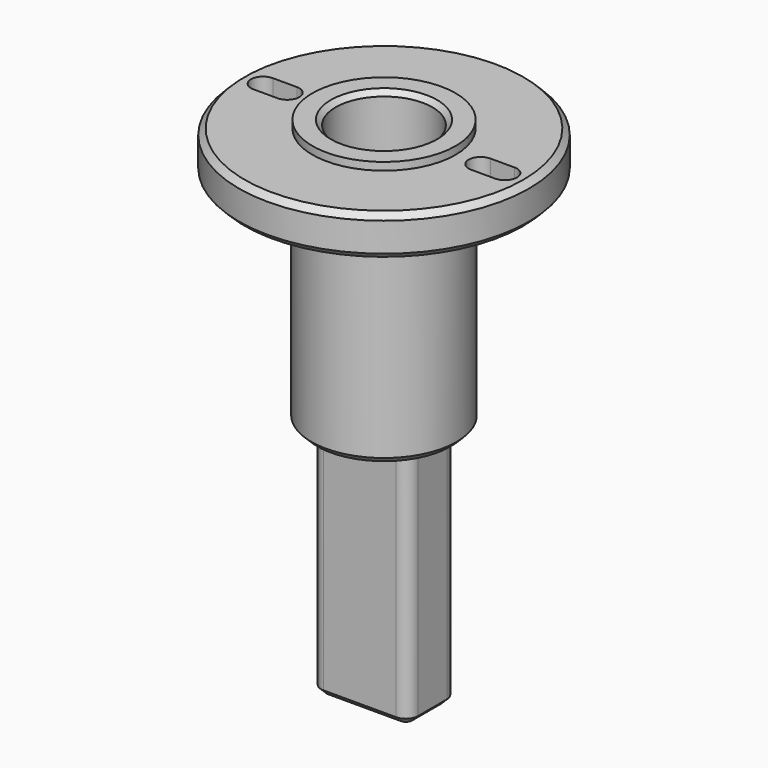
from build123d import *

# Parameters (mm, degrees)
F0_R           = 19.05
F1_DEPTH       = 5.334
F2_R           = 9.398
F3_DEPTH       = 1.016
F4_R           = 9.525
F5_DEPTH       = 28.575
F6_W           = 12.7
F6_H           = 7.9248
F7_DEPTH       = 31.75
F9_D           = 12.7
F9_DEPTH       = 28.575
F9_CSINK_D     = 13.97
F9_CSINK_ANGLE = 90
F9_TIP         = 3.8154649308
F10_SIZE       = 0.762
F12_D          = 2.3876
F14_D          = 2.4892
F14_DEPTH      = 14.732
F14_TIP        = 0.7478311264
F16_D          = 3.175
F16_DEPTH      = 9.525
F16_TIP        = 0.9538662327
F18_D          = 4.3688
F18_DEPTH      = 1.905
F18_START      = 32.1342766
F18_TIP        = 1.3125199362
F20_DEPTH      = 3.81
F21_R          = 1.5748
F22_SIZE       = 0.762


# Not quite as in the source:
# - a length typed as a fraction of an inch, garbled in the dataset ("3 / 203.2 mm" for 3/8 in), is restored


with BuildPart() as f1:
    # F0 (on Top) → F1 (new body)
    with BuildSketch(Plane.XY):
        Circle(F0_R)
    extrude(amount=F1_DEPTH)

    # F2 (on face) → F3 (join)
    with BuildSketch(Plane.XY.offset(5.334)):
        Circle(F2_R)
    extrude(amount=F3_DEPTH)

    # F4 (on face) → F5 (join)
    with BuildSketch(Plane(origin=(0, 0, 0), x_dir=(1, 0, 0), z_dir=(0, 0, -1))):
        Circle(F4_R)
    extrude(amount=F5_DEPTH)

    # F6 (on face) → F7 (join)
    with BuildSketch(Plane(origin=(0, 0, -28.575), x_dir=(1, 0, 0), z_dir=(0, 0, -1))):
        Rectangle(F6_W, F6_H)
    extrude(amount=F7_DEPTH)

    # F9
    with Locations(Plane.XY.offset(6.35)):
        with Locations((0, 0)):
            CounterSinkHole(F9_D / 2, F9_CSINK_D / 2, depth=F9_DEPTH, counter_sink_angle=F9_CSINK_ANGLE)
            with Locations((0, 0, -(F9_DEPTH + F9_TIP / 2))):  # 118° drill point
                Cone(0, F9_D / 2, F9_TIP, mode=Mode.SUBTRACT)

    # F10
    f10_edges = [f1.edges().sort_by_distance(p)[0] for p in [
        (-9.525, 0, -28.575),
        (-19.05, 0, 0),
        (-19.05, 0, 5.334),
    ]]
    chamfer(f10_edges, length=F10_SIZE)

    # F12 (through all)
    with Locations(Plane(origin=(0, 0, -60.325), x_dir=(1, 0, 0), z_dir=(0, 0, -1))):
        with Locations((2.4892, -0.7874), (-2.4892, -0.7874)):
            Hole(F12_D / 2)

    # F14
    with Locations(Plane(origin=(0, 0, -60.325), x_dir=(1, 0, 0), z_dir=(0, 0, -1))):
        with Locations((2.4892, -0.7874), (-2.4892, -0.7874)):
            Hole(F14_D / 2, depth=F14_DEPTH)
            with Locations((0, 0, -(F14_DEPTH + F14_TIP / 2))):  # 118° drill point
                Cone(0, F14_D / 2, F14_TIP, mode=Mode.SUBTRACT)

    # F16
    with Locations(Plane(origin=(0, 0, -60.325), x_dir=(1, 0, 0), z_dir=(0, 0, -1))):
        with Locations((2.4892, -0.7874), (-2.4892, -0.7874)):
            Hole(F16_D / 2, depth=F16_DEPTH)
            with Locations((0, 0, -(F16_DEPTH + F16_TIP / 2))):  # 118° drill point
                Cone(0, F16_D / 2, F16_TIP, mode=Mode.SUBTRACT)

    # F18
    # its depths count from where the whole tool has entered the part; down to there all is cleared
    with Locations(Plane.XY.offset(6.35)):
        with Locations((2.4892, 0.7874), (-2.4892, 0.7874)):
            Hole(F18_D / 2, depth=F18_START)
    with Locations(Plane.XY.offset(6.35).offset(-F18_START)):
        with Locations((2.4892, 0.7874), (-2.4892, 0.7874)):
            Hole(F18_D / 2, depth=F18_DEPTH)
            with Locations((0, 0, -(F18_DEPTH + F18_TIP / 2))):  # 118° drill point
                Cone(0, F18_D / 2, F18_TIP, mode=Mode.SUBTRACT)

    # F19 (on face) → F20 (cut)
    with BuildSketch(Plane.XY.offset(5.334)):
        with BuildLine():
            ThreePointArc((15.875, 1.5875), (14.7524679849, 1.1225320151), (14.2875, 0))
            ThreePointArc((14.2875, 0), (14.7524679849, -1.1225320151), (15.875, -1.5875))
            ThreePointArc((15.875, -1.5875), (16.9975320151, -1.1225320151), (17.4625, 0))
            ThreePointArc((17.4625, 0), (16.9975320151, 1.1225320151), (15.875, 1.5875))
        make_face()
        with BuildLine():
            ThreePointArc((12.7, -1.5875), (13.8225320151, -1.1225320151), (14.2875, 0))
            ThreePointArc((14.2875, 0), (13.8225320151, 1.1225320151), (12.7, 1.5875))
            Line((12.7, 1.5875), (12.7, -1.5875))
        make_face()
        with BuildLine():
            ThreePointArc((12.7, 1.5875), (13.8225320151, 1.1225320151), (14.2875, 0))
            ThreePointArc((14.2875, 0), (14.7524679849, 1.1225320151), (15.875, 1.5875))
            Line((15.875, 1.5875), (12.7, 1.5875))
        make_face()
        with BuildLine():
            Line((12.7, -1.5875), (12.7, 1.5875))
            ThreePointArc((12.7, 1.5875), (11.1125, 0), (12.7, -1.5875))
        make_face()
        with BuildLine():
            ThreePointArc((15.875, -1.5875), (14.7524679849, -1.1225320151), (14.2875, 0))
            ThreePointArc((14.2875, 0), (13.8225320151, -1.1225320151), (12.7, -1.5875))
            Line((12.7, -1.5875), (15.875, -1.5875))
        make_face()
        with BuildLine():
            ThreePointArc((-12.7, -1.5875), (-11.5774679849, -1.1225320151), (-11.1125, 0))
            ThreePointArc((-11.1125, 0), (-11.5774679849, 1.1225320151), (-12.7, 1.5875))
            ThreePointArc((-12.7, 1.5875), (-13.8225320151, 1.1225320151), (-14.2875, 0))
            ThreePointArc((-14.2875, 0), (-13.8225320151, -1.1225320151), (-12.7, -1.5875))
        make_face()
        with BuildLine():
            Line((-15.875, -1.5875), (-12.7, -1.5875))
            ThreePointArc((-12.7, -1.5875), (-13.8225320151, -1.1225320151), (-14.2875, 0))
            ThreePointArc((-14.2875, 0), (-14.7524679849, -1.1225320151), (-15.875, -1.5875))
        make_face()
        with BuildLine():
            ThreePointArc((-14.2875, 0), (-13.8225320151, 1.1225320151), (-12.7, 1.5875))
            Line((-12.7, 1.5875), (-15.875, 1.5875))
            ThreePointArc((-15.875, 1.5875), (-14.7524679849, 1.1225320151), (-14.2875, 0))
        make_face()
        with BuildLine():
            ThreePointArc((-15.875, -1.5875), (-14.7524679849, -1.1225320151), (-14.2875, 0))
            ThreePointArc((-14.2875, 0), (-14.7524679849, 1.1225320151), (-15.875, 1.5875))
            ThreePointArc((-15.875, 1.5875), (-17.4625, 0), (-15.875, -1.5875))
        make_face()
    extrude(amount=-F20_DEPTH, mode=Mode.SUBTRACT)

    # F21
    f21_edges = [f1.edges().sort_by_distance(p)[0] for p in [
        (6.35, 3.9624, -44.45),
        (6.35, -3.9624, -44.45),
        (-6.35, -3.9624, -44.45),
        (-6.35, 3.9624, -44.45),
    ]]
    fillet(f21_edges, radius=F21_R)

    # F22
    f22_edges = [f1.edges().sort_by_distance(p)[0] for p in [
        (6.35, 0, -60.325),
        (5.888752, -3.501152, -60.325),
        (0, -3.9624, -60.325),
        (-6.35, 0, -60.325),
        (-5.888752, -3.501152, -60.325),
        (0, 3.9624, -60.325),
        (5.888752, 3.501152, -60.325),
    ]]
    chamfer(f22_edges, length=F22_SIZE)


solid = f1.part
